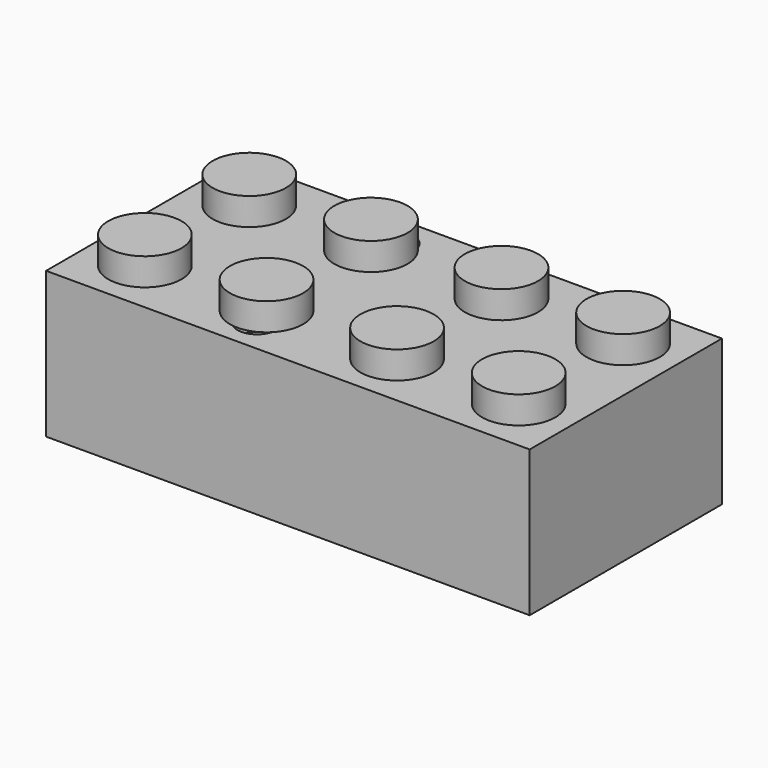
from build123d import *

# Parameters (mm, degrees)
F0_W      = 31.8
F0_H      = 15.8
F1_DEPTH  = 4.8
F2_W      = 29.4
F2_H      = 13.4
F3_DEPTH  = 8.4
F4_R      = 2.409
F5_DEPTH  = 1.8
F6_R      = 1.3
F7_DEPTH  = 1.2
F8_R      = 2.409
F9_DEPTH  = 8.4
F10_W     = 0.3
F10_H     = 0.6
F11_DEPTH = 8.4
F12_W     = 0.6
F12_H     = 0.3
F13_DEPTH = 8.4
F14_W     = 0.8
F14_H     = 3.4696710694
F15_DEPTH = 6.4


with BuildPart() as f1:
    # F0 (on Top) → F1 (new body, symmetric)
    with BuildSketch(Plane.XY):
        Rectangle(F0_W, F0_H)
    extrude(amount=F1_DEPTH, both=True)

    # F2 (on face) → F3 (cut)
    with BuildSketch(Plane(origin=(0, 0, -4.8), x_dir=(1, 0, 0), z_dir=(0, 0, -1))):
        Rectangle(F2_W, F2_H)
    extrude(amount=-F3_DEPTH, mode=Mode.SUBTRACT)

    # F4 (on face) → F5 (join)
    with BuildSketch(Plane.XY.offset(4.8)):
        with Locations((-12.291, 4.2910612803)):
            Circle(F4_R)
        with Locations((12.291, 4.2910612803)):
            Circle(F4_R)
        with Locations((-12.291, -4.2910612803)):
            Circle(F4_R)
        with Locations((12.291, -4.2910612803)):
            Circle(F4_R)
        with Locations((-4.291, 4.2910612803)):
            Circle(F4_R)
        with Locations((4.291, 4.2910612803)):
            Circle(F4_R)
        with Locations((-4.291, -4.2910612803)):
            Circle(F4_R)
        with Locations((4.291, -4.2910612803)):
            Circle(F4_R)
    extrude(amount=F5_DEPTH)

    # F6 (on face) → F7 (cut)
    with BuildSketch(Plane(origin=(0, 0, 3.6), x_dir=(1, 0, 0), z_dir=(0, 0, -1))):
        with Locations((-11.8301756735, 4)):
            Circle(F6_R)
        with Locations((-3.8301756735, 5.6396185296)):
            Circle(F6_R)
        with Locations((4, 4)):
            Circle(F6_R)
        with Locations((12, 4)):
            Circle(F6_R)
        with Locations((-11.8301756735, -4)):
            Circle(F6_R)
        with Locations((-3.8301756735, -5.6396185296)):
            Circle(F6_R)
        with Locations((4, -4)):
            Circle(F6_R)
        with Locations((12, -4)):
            Circle(F6_R)
    extrude(amount=-F7_DEPTH, mode=Mode.SUBTRACT)

    # F8 (on face) → F9 (join, through all)
    with BuildSketch(Plane(origin=(0, 0, 3.6), x_dir=(1, 0, 0), z_dir=(0, 0, -1))):
        Circle(F8_R)
    extrude(amount=F9_DEPTH)

    # F10 (on face) → F11 (join, through all)
    with BuildSketch(Plane(origin=(0, 0, 3.6), x_dir=(1, 0, 0), z_dir=(0, 0, -1))):
        with Locations((-14.55, 4)):
            Rectangle(F10_W, F10_H)
        with Locations((-14.55, -4)):
            Rectangle(F10_W, F10_H)
        with Locations((14.55, 4)):
            Rectangle(F10_W, F10_H)
        with Locations((14.55, -4)):
            Rectangle(F10_W, F10_H)
    extrude(amount=F11_DEPTH)

    # F12 (on face) → F13 (join, through all)
    with BuildSketch(Plane(origin=(0, 0, 3.6), x_dir=(1, 0, 0), z_dir=(0, 0, -1))):
        with Locations((-11.8301756735, 6.55)):
            Rectangle(F12_W, F12_H)
        with Locations((-3.8301756735, 6.55)):
            Rectangle(F12_W, F12_H)
        with Locations((4, 6.55)):
            Rectangle(F12_W, F12_H)
        with Locations((12.3396486531, 6.55)):
            Rectangle(F12_W, F12_H)
        with Locations((-3.8301756735, -6.55)):
            Rectangle(F12_W, F12_H)
        with Locations((-11.8301756735, -6.55)):
            Rectangle(F12_W, F12_H)
        with Locations((4, -6.55)):
            Rectangle(F12_W, F12_H)
        with Locations((12.3396486531, -6.55)):
            Rectangle(F12_W, F12_H)
    extrude(amount=F13_DEPTH)

    # F14 (on face) → F15 (join)
    with BuildSketch(Plane(origin=(0, 0, 3.6), x_dir=(1, 0, 0), z_dir=(0, 0, -1))):
        with Locations((0, 4.9651644653)):
            Rectangle(F14_W, F14_H)
        with Locations((0, -4.9651644653)):
            Rectangle(F14_W, F14_H)
    extrude(amount=F15_DEPTH)


solid = f1.part
